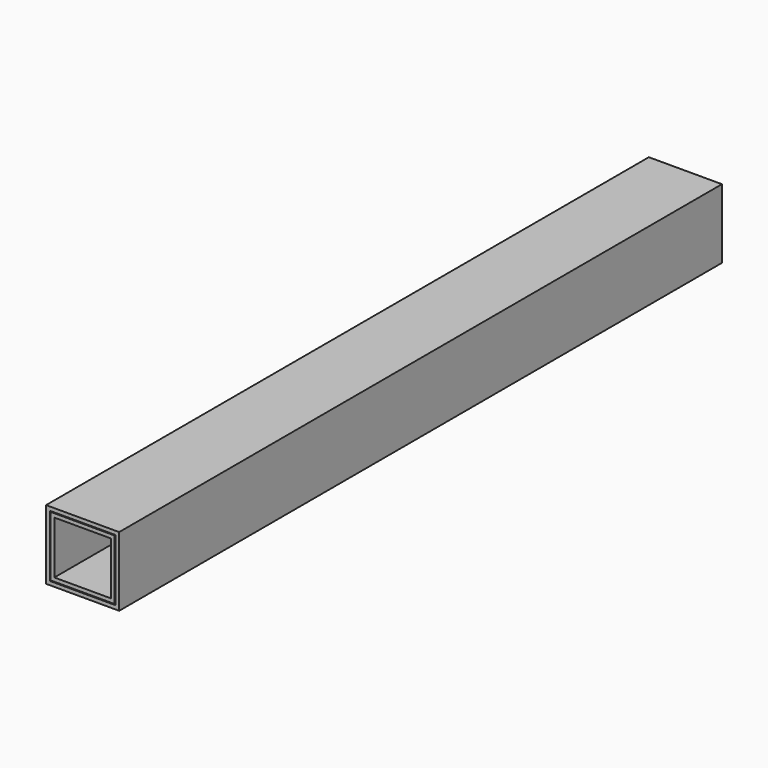
from build123d import *

# Parameters (mm, degrees)
F0_W     = 17
F0_H     = 16
F0_W_2   = 15
F0_H_2   = 14
F1_DEPTH = 200
F2_DEPTH = 1
F0_W_3   = 19.4
F0_H_3   = 18.4
F0_W_4   = 17.4
F0_H_4   = 16.4
F3_DEPTH = 200
F4_DEPTH = 1
F5_DEPTH = 10


with BuildPart() as f1:
    # F0 (on Front) → F1 (new body)
    with BuildSketch(Plane.XZ):
        Rectangle(F0_W, F0_H)
        Rectangle(F0_W_2, F0_H_2, mode=Mode.SUBTRACT)
    extrude(amount=F1_DEPTH)

    # F0 (on Front) → F2 (join)
    with BuildSketch(Plane.XZ):
        Rectangle(F0_W_2, F0_H_2)
    extrude(amount=F2_DEPTH)


with BuildPart() as f3:
    # F0 (on Front) → F3 (new body)
    with BuildSketch(Plane.XZ):
        Rectangle(F0_W_3, F0_H_3)
        Rectangle(F0_W_4, F0_H_4, mode=Mode.SUBTRACT)
    extrude(amount=F3_DEPTH)

    # F0 (on Front) → F4 (join)
    with BuildSketch(Plane.XZ):
        Rectangle(F0_W_4, F0_H_4)
        Rectangle(F0_W, F0_H, mode=Mode.SUBTRACT)
        Rectangle(F0_W, F0_H)
        Rectangle(F0_W_2, F0_H_2, mode=Mode.SUBTRACT)
        Rectangle(F0_W_2, F0_H_2)
    extrude(amount=F4_DEPTH)


with BuildPart() as f5:
    # F0 (on Front) → F5 (new body)
    with BuildSketch(Plane.XZ):
        Rectangle(F0_W, F0_H)
        Rectangle(F0_W_2, F0_H_2, mode=Mode.SUBTRACT)
    extrude(amount=F5_DEPTH)


solid = Compound([f1.part, f3.part, f5.part])
